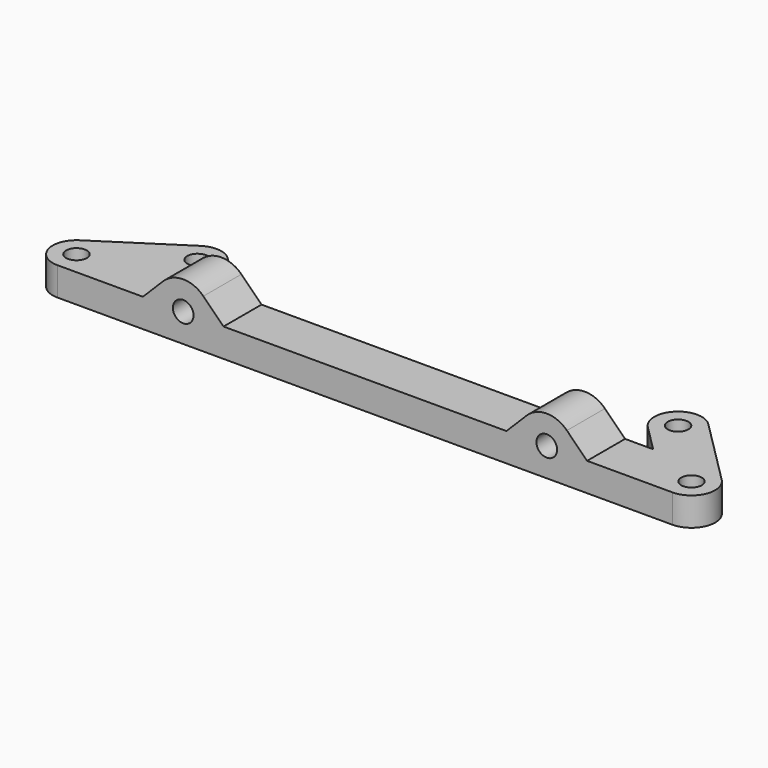
from build123d import *

# Parameters (mm, degrees)
F0_R     = 1.7272
F1_DEPTH = 4.7625
F3_DEPTH = 7.9375
F4_R     = 1.7272
F5_DEPTH = 7.9375


with BuildPart() as f1:
    # F0 (on Top) → F1 (new body)
    with BuildSketch(Plane.XY):
        with BuildLine():
            Line((-4.4502401135, 4.4502401135), (0, 0))
            Line((0, 0), (-79.7381539824, 0))
            Line((-79.7381539824, 0), (-77.6839886087, 1.3305217617))
            ThreePointArc((-77.6839886087, 1.3305217617), (-76.5105259182, 6.8191407537), (-81.9991449101, 7.9926034442))
            Line((-81.9991449101, 7.9926034442), (-95.3233082751, -0.6377091588))
            ThreePointArc((-95.3233082751, -0.6377091588), (-96.9717152071, -5.0936740472), (-93.1657301243, -7.9375))
            Line((-93.1657301243, -7.9375), (9.5814100757, -7.9375))
            ThreePointArc((9.5814100757, -7.9375), (13.2480569703, -5.4875248722), (12.3877401135, -1.1624199622))
            Line((12.3877401135, -1.1624199622), (1.1624199622, 10.0629001892))
            ThreePointArc((1.1624199622, 10.0629001892), (-4.4502401135, 10.0629001892), (-4.4502401135, 4.4502401135))
        make_face()
        with Locations((-93.1657301243, -3.96875)):
            Circle(F0_R, mode=Mode.SUBTRACT)
        with Locations((9.5814100757, -3.96875)):
            Circle(F0_R, mode=Mode.SUBTRACT)
        with Locations((-79.8415667594, 4.661562603)):
            Circle(F0_R, mode=Mode.SUBTRACT)
        with Locations((-1.6439100757, 7.2565701513)):
            Circle(F0_R, mode=Mode.SUBTRACT)
    extrude(amount=F1_DEPTH)

    # F2 (on face) → F3 (join, through all)
    with BuildSketch(Plane.XZ.offset(7.9375)):
        with BuildLine():
            Line((-78.8949317151, 4.7625), (-72.1597396243, 4.7625))
            Line((-72.1597396243, 4.7625), (-65.4245475335, 4.7625))
            Line((-65.4245475335, 4.7625), (-68.7921435789, 8.1300960454))
            ThreePointArc((-68.7921435789, 8.1300960454), (-72.1597396243, 9.525), (-75.5273356697, 8.1300960454))
            Line((-75.5273356697, 8.1300960454), (-78.8949317151, 4.7625))
        make_face()
        with BuildLine():
            Line((-18.1597725151, 4.7625), (-11.4245804243, 4.7625))
            Line((-11.4245804243, 4.7625), (-4.6893883335, 4.7625))
            Line((-4.6893883335, 4.7625), (-8.0569843789, 8.1300960454))
            ThreePointArc((-8.0569843789, 8.1300960454), (-11.4245804243, 9.525), (-14.7921764697, 8.1300960454))
            Line((-14.7921764697, 8.1300960454), (-18.1597725151, 4.7625))
        make_face()
    extrude(amount=-F3_DEPTH)

    # F4 (on face) → F5 (cut, through all)
    with BuildSketch(Plane.XZ.offset(7.9375)):
        with Locations((-72.1597396243, 4.7625)):
            Circle(F4_R)
        with Locations((-11.4245804243, 4.7625)):
            Circle(F4_R)
    extrude(amount=-F5_DEPTH, mode=Mode.SUBTRACT)


solid = f1.part
